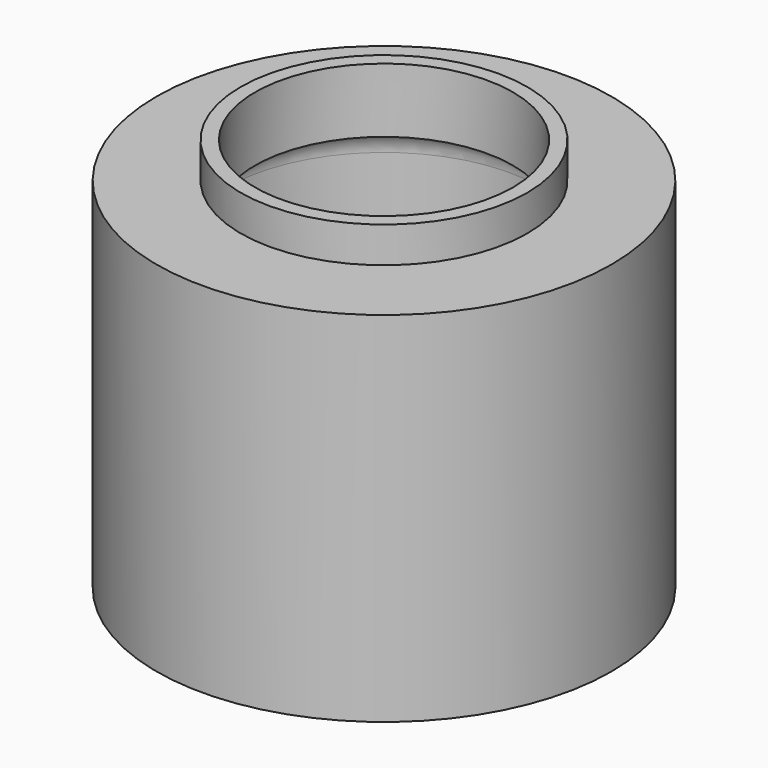
from build123d import *

# Parameters (mm, degrees)
F0_R     = 15.875
F0_R_2   = 9
F1_DEPTH = 25
F2_R     = 10
F2_R_2   = 9
F3_DEPTH = 2.5
F4_R     = 11
F4_R_2   = 9
F5_DEPTH = 23
F6_R     = 1.99999
F7_DEPTH = 2.5


# Not quite as in the source:
# - a fillet or chamfer is up to 0.001 mm smaller than in the source, because OpenCascade refuses the exact size


with BuildPart() as f1:
    # F0 (on Top) → F1 (new body)
    with BuildSketch(Plane.XY):
        Circle(F0_R)
        Circle(F0_R_2, mode=Mode.SUBTRACT)
    extrude(amount=F1_DEPTH)

    # F2 (on face) → F3 (join)
    with BuildSketch(Plane.XY.offset(25)):
        Circle(F2_R)
        Circle(F2_R_2, mode=Mode.SUBTRACT)
    extrude(amount=F3_DEPTH)

    # F4 (on face) → F5 (cut)
    with BuildSketch(Plane(origin=(0, 0, 0), x_dir=(1, 0, 0), z_dir=(0, 0, -1))):
        Circle(F4_R)
        Circle(F4_R_2, mode=Mode.SUBTRACT)
    extrude(amount=-F5_DEPTH, mode=Mode.SUBTRACT)

    # F6 (radius 2 in the source; OpenCascade refuses exactly that, so slightly less here)
    f6_edges = [f1.edges().sort_by_distance(p)[0] for p in [
        (-11, 0, 23),
    ]]
    fillet(f6_edges, radius=F6_R)

    # F2 (on face) → F7 (join)
    with BuildSketch(Plane.XY.offset(25)):
        Circle(F2_R)
        Circle(F2_R_2, mode=Mode.SUBTRACT)
    extrude(amount=F7_DEPTH)


solid = f1.part
